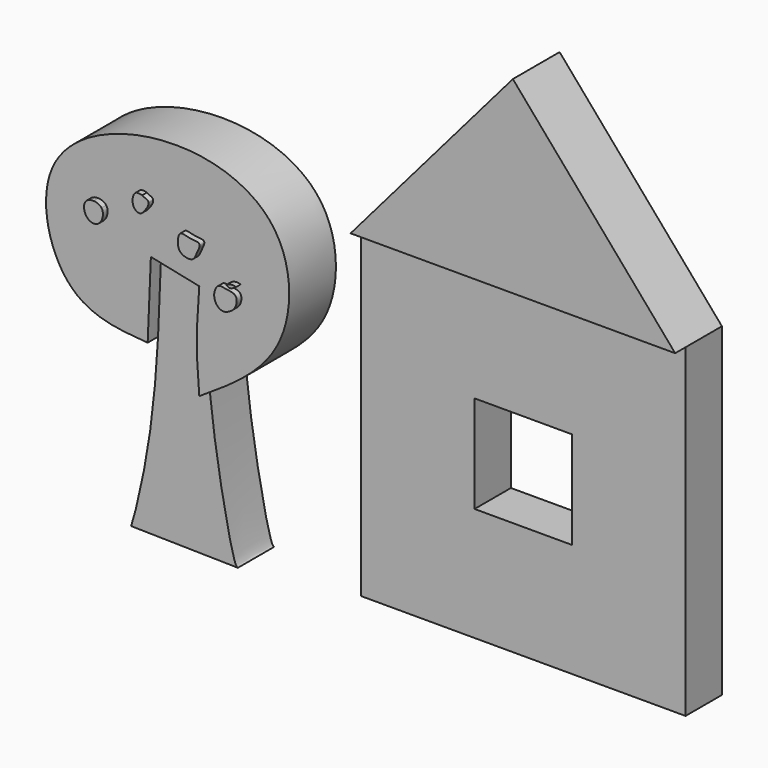
from build123d import *

# Parameters (mm, degrees)
F0_W     = 15
F0_H     = 15
F1_DEPTH = 7
F2_DEPTH = 9
F3_DEPTH = 7
F4_DEPTH = 9
F5_DEPTH = 9.9


with BuildPart() as f1:
    # F0 (on Front) → F1 (new body)
    with BuildSketch(Plane.XZ):
        Polygon((25, -5.523831), (25, 25), (-25, 25), (-25, -25), (25, -25), (25, -13.455487), align=None)
        Rectangle(F0_W, F0_H, mode=Mode.SUBTRACT)
    extrude(amount=F1_DEPTH)

    # F0 (on Front) → F2 (join)
    with BuildSketch(Plane.XZ):
        Polygon((-25, 25), (25, 25), (0, 54.053254), align=None)
    extrude(amount=F2_DEPTH)


with BuildPart() as f3:
    # F0 (on Front) → F3 (new body)
    with BuildSketch(Plane.XZ):
        with BuildLine():
            Line((-48.306216, 10.251479), (-55.761836, 11.804733))
            add(Edge.make_bspline(
                [(-55.761836, 11.804733), (-55.844109, 9.412009), (-55.954941, 6.188702), (-56.181615, 1.334385), (-56.255277, 0)],
                knots=[0, 0, 0, 0, 0.253646, 0.341694, 0.341694, 0.341694, 0.341694], degree=3))
            add(Edge.make_bspline(
                [(-56.255277, 0), (-56.515152, -4.70766), (-57.39622, -15.967553), (-60.280233, -27.042113), (-60.421601, -27.026627)],
                knots=[0.341694, 0.341694, 0.341694, 0.341694, 0.652324, 0.950274, 0.950274, 0.950274, 0.950274], degree=3))
            Line((-60.421601, -27.026627), (-43.957103, -27.337279))
            add(Edge.make_bspline(
                [(-48.306216, -4.659764), (-47.486241, -12.968249), (-44.822625, -27.013395), (-44.051256, -27.302046), (-43.957103, -27.337279)],
                knots=[0.415584, 0.415584, 0.415584, 0.415584, 0.928666, 1, 1, 1, 1], degree=3))
            add(Edge.make_bspline(
                [(-48.306216, 10.251479), (-48.638295, 6.160688), (-48.970374, 2.069897), (-48.306216, -4.659764)],
                knots=[0, 0, 0, 0, 0.415584, 0.415584, 0.415584, 0.415584], degree=3))
        make_face()
    extrude(amount=F3_DEPTH)

    # F0 (on Front) → F4 (join)
    with BuildSketch(Plane.XZ):
        with BuildLine():
            add(Edge.make_bspline(
                [(-55.761836, 11.804733), (-55.844109, 9.412009), (-55.954941, 6.188702), (-56.181615, 1.334385), (-56.255277, 0)],
                knots=[0, 0, 0, 0, 0.253646, 0.341694, 0.341694, 0.341694, 0.341694], degree=3))
            Line((-55.761836, 11.804733), (-48.306216, 10.251479))
            add(Edge.make_bspline(
                [(-48.306216, 10.251479), (-48.638295, 6.160688), (-48.970374, 2.069897), (-48.306216, -4.659764)],
                knots=[0, 0, 0, 0, 0.415584, 0.415584, 0.415584, 0.415584], degree=3))
            add(Edge.make_bspline(
                [(-56.255277, 0), (-60.629021, 0.325235), (-69.925979, 1.016565), (-75.055072, 21.903906), (-53.592436, 30.741506), (-33.999012, 24.583978), (-33.636713, 4.765701), (-43.34652, -1.473054), (-48.306216, -4.659764)],
                knots=[0, 0, 0, 0, 0.145761, 0.309833, 0.49303, 0.668184, 0.830511, 1, 1, 1, 1], degree=3))
        make_face()
        with BuildLine():
            add(Edge.make_bspline(
                [(-43.427911, 11.804733), (-43.924175, 11.887406), (-44.886479, 12.19435), (-45.625923, 9.997869), (-44.34338, 8.395903), (-42.894572, 8.843332), (-41.811672, 9.792412), (-41.702126, 11.671268), (-42.892401, 11.715523), (-43.427911, 11.804733)],
                knots=[0, 0, 0, 0, 0.132419, 0.290195, 0.444053, 0.577382, 0.717505, 0.857109, 1, 1, 1, 1], degree=3))
        make_face(mode=Mode.SUBTRACT)
        with BuildLine():
            add(Edge.make_bspline(
                [(-43.427911, 12.387617), (-43.249994, 12.254753), (-42.84739, 11.954097), (-42.276843, 12.334602), (-41.958429, 12.546957)],
                knots=[0, 0, 0, 0, 0.441913, 1, 1, 1, 1], degree=3))
            add(Edge.make_bspline(
                [(-43.427911, 12.387617), (-43.256797, 12.487744), (-42.902567, 12.695021), (-42.154906, 12.672184), (-42.00987, 12.579744), (-41.958429, 12.546957)],
                knots=[0, 0, 0, 0, 0.37618, 0.778745, 1, 1, 1, 1], degree=3))
        make_face(mode=Mode.SUBTRACT)
        with BuildLine():
            add(Edge.make_bspline(
                [(-62.650077, 16.571494), (-62.901276, 16.915807), (-63.38094, 17.102787), (-63.860662, 17.12387)],
                knots=[0, 0, 0, 0, 0.138546, 0.138546, 0.138546, 0.138546], degree=3))
            add(Edge.make_bspline(
                [(-63.860662, 17.12387), (-64.277854, 17.142205), (-65.562812, 16.812272), (-65.337126, 14.266247), (-62.811091, 13.655118), (-62.176873, 15.922883), (-62.650077, 16.571494)],
                knots=[0.138546, 0.138546, 0.138546, 0.138546, 0.259033, 0.50961, 0.739009, 1, 1, 1, 1], degree=3))
        make_face(mode=Mode.SUBTRACT)
        with BuildLine():
            add(Edge.make_bspline(
                [(-49.032278, 16.886169), (-49.640072, 16.984131), (-50.68548, 17.481857), (-50.966268, 15.772906), (-50.710337, 14.225715), (-48.497249, 13.809135), (-48.071119, 15.105466), (-47.06323, 16.913458), (-48.41982, 16.787455), (-49.032278, 16.886169)],
                knots=[0, 0, 0, 0, 0.143813, 0.278051, 0.422275, 0.576903, 0.711141, 0.855083, 1, 1, 1, 1], degree=3))
        make_face(mode=Mode.SUBTRACT)
        with BuildLine():
            add(Edge.make_bspline(
                [(-56.357041, 20.34012), (-56.780966, 20.422877), (-57.735343, 20.609186), (-58.092267, 18.371826), (-56.596495, 17.300513), (-55.884236, 18.475069), (-55.493552, 19.119328)],
                knots=[0, 0, 0, 0, 0.218254, 0.491352, 0.721, 1, 1, 1, 1], degree=3))
            add(Edge.make_bspline(
                [(-55.493552, 19.119328), (-55.418936, 19.389647), (-55.256013, 19.979885), (-56.160313, 20.110778), (-56.357041, 20.34012)],
                knots=[0, 0, 0, 0, 0.296408, 0.647204, 0.647204, 0.647204, 0.647204], degree=3))
        make_face(mode=Mode.SUBTRACT)
    extrude(amount=F4_DEPTH)

    # F0 (on Front) → F5 (join)
    with BuildSketch(Plane.XZ):
        with BuildLine():
            add(Edge.make_bspline(
                [(-43.427911, 11.804733), (-43.924175, 11.887406), (-44.886479, 12.19435), (-45.625923, 9.997869), (-44.34338, 8.395903), (-42.894572, 8.843332), (-41.811672, 9.792412), (-41.702126, 11.671268), (-42.892401, 11.715523), (-43.427911, 11.804733)],
                knots=[0, 0, 0, 0, 0.132419, 0.290195, 0.444053, 0.577382, 0.717505, 0.857109, 1, 1, 1, 1], degree=3))
        make_face()
        with BuildLine():
            add(Edge.make_bspline(
                [(-49.032278, 16.886169), (-49.640072, 16.984131), (-50.68548, 17.481857), (-50.966268, 15.772906), (-50.710337, 14.225715), (-48.497249, 13.809135), (-48.071119, 15.105466), (-47.06323, 16.913458), (-48.41982, 16.787455), (-49.032278, 16.886169)],
                knots=[0, 0, 0, 0, 0.143813, 0.278051, 0.422275, 0.576903, 0.711141, 0.855083, 1, 1, 1, 1], degree=3))
        make_face()
        with BuildLine():
            add(Edge.make_bspline(
                [(-55.493552, 19.119328), (-55.418936, 19.389647), (-55.256013, 19.979885), (-56.160313, 20.110778), (-56.357041, 20.34012)],
                knots=[0, 0, 0, 0, 0.296408, 0.647204, 0.647204, 0.647204, 0.647204], degree=3))
            add(Edge.make_bspline(
                [(-56.357041, 20.34012), (-56.780966, 20.422877), (-57.735343, 20.609186), (-58.092267, 18.371826), (-56.596495, 17.300513), (-55.884236, 18.475069), (-55.493552, 19.119328)],
                knots=[0, 0, 0, 0, 0.218254, 0.491352, 0.721, 1, 1, 1, 1], degree=3))
        make_face()
        with BuildLine():
            add(Edge.make_bspline(
                [(-63.860662, 17.12387), (-64.277854, 17.142205), (-65.562812, 16.812272), (-65.337126, 14.266247), (-62.811091, 13.655118), (-62.176873, 15.922883), (-62.650077, 16.571494)],
                knots=[0.138546, 0.138546, 0.138546, 0.138546, 0.259033, 0.50961, 0.739009, 1, 1, 1, 1], degree=3))
            add(Edge.make_bspline(
                [(-62.650077, 16.571494), (-62.901276, 16.915807), (-63.38094, 17.102787), (-63.860662, 17.12387)],
                knots=[0, 0, 0, 0, 0.138546, 0.138546, 0.138546, 0.138546], degree=3))
        make_face()
        with BuildLine():
            add(Edge.make_bspline(
                [(-43.427911, 12.387617), (-43.256797, 12.487744), (-42.902567, 12.695021), (-42.154906, 12.672184), (-42.00987, 12.579744), (-41.958429, 12.546957)],
                knots=[0, 0, 0, 0, 0.37618, 0.778745, 1, 1, 1, 1], degree=3))
            add(Edge.make_bspline(
                [(-43.427911, 12.387617), (-43.249994, 12.254753), (-42.84739, 11.954097), (-42.276843, 12.334602), (-41.958429, 12.546957)],
                knots=[0, 0, 0, 0, 0.441913, 1, 1, 1, 1], degree=3))
        make_face()
    extrude(amount=F5_DEPTH)


solid = Compound([f1.part, f3.part])
